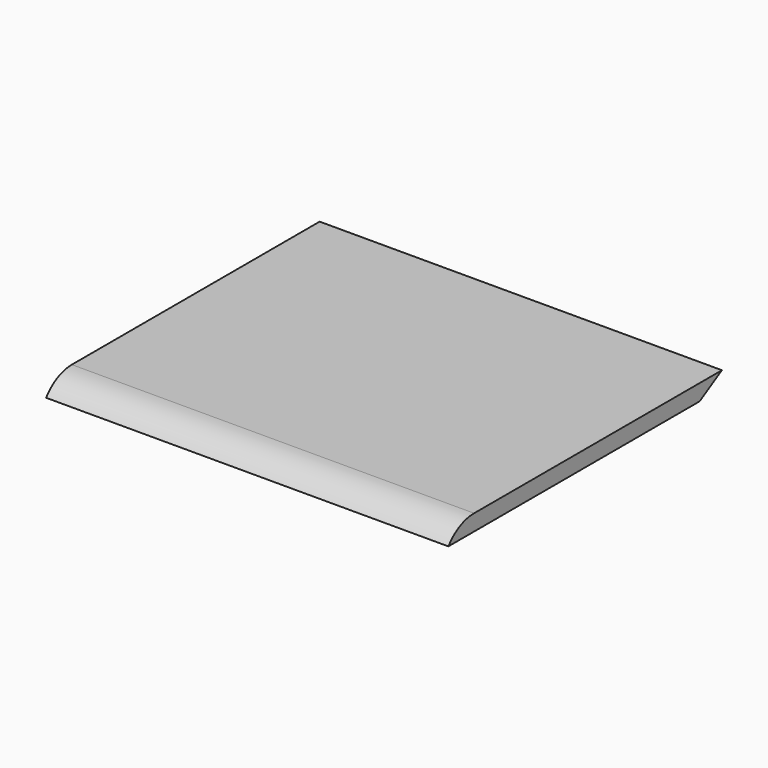
from build123d import *

# Parameters (mm, degrees)
F0_W        = 50
F0_H        = 42.5
F1_DEPTH    = 2
F2_SIZE2    = 3.464092
F2_SIZE     = 1.99999
F3_T1_DEPTH = 70


# Not quite as in the source:
# - a fillet or chamfer that OpenCascade refuses, or shapes differently, is made with other operations: its cross-section is extruded or revolved along the edge and cut away or added
# - a fillet or chamfer is up to 0.001 mm smaller than in the source, because OpenCascade refuses the exact size


with BuildPart() as f1:
    # F0 (on Top) → F1 (new body)
    with BuildSketch(Plane.XY):
        with Locations((-25, -21.25)):
            Rectangle(F0_W, F0_H)
    extrude(amount=F1_DEPTH)

    # F2 (size 2 and 3.4641016151 in the source; OpenCascade refuses exactly that, so slightly less here)
    f2_edges = [f1.edges().sort_by_distance(p)[0] for p in [
        (-25, 0, 0),
    ]]
    f2_side = f1.faces().sort_by_distance((-25, 0, 1))[0]
    chamfer(f2_edges, length=F2_SIZE, length2=F2_SIZE2, reference=f2_side)

    # F3: fillet of radius 5 on 1 edges, made by hand

    # F3_s2 → F3_t1 (cut)
    with BuildSketch(Plane.YZ.offset(-60)):
        with BuildLine():
            ThreePointArc((-38.5, 2), (-40.7360679775, 1.472135955), (-42.5, 0))
            Line((-42.5, 0), (-42.5, 2))
            Line((-42.5, 2), (-38.5, 2))
        make_face()
    extrude(amount=F3_T1_DEPTH, mode=Mode.SUBTRACT)


solid = f1.part
